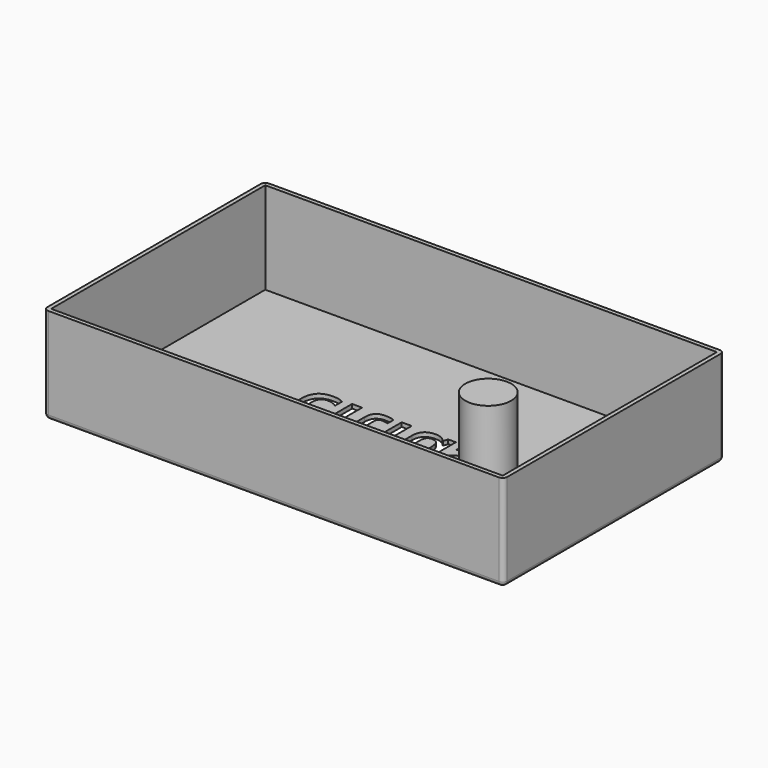
from build123d import *

# Parameters (mm, degrees)
F0_W         = 100
F0_H         = 60
F1_DEPTH     = 0.9
F2_W         = 98.2
F2_H         = 0.9
F3_DEPTH     = 20
F4_TEXT_SIZE = 14.6002053154
F5_DEPTH     = 2
F6_R         = 5
F7_DEPTH     = 25
F8_R         = 1
F8_2_R       = 1


# Not quite as in the source:
# - Text() gives the source's letters only with a copy of the font that has no kerning and outlines rounded to 1/6400 em; it was checked with that copy


with BuildPart() as f1:
    # F0 (on Top) → F1 (new body)
    with BuildSketch(Plane.XY):
        with Locations((2.3630317301, -8.3058337704)):
            Rectangle(F0_W, F0_H)
    extrude(amount=F1_DEPTH)

    # F2 (on face) → F3 (join)
    with BuildSketch(Plane.XY.offset(0.9)):
        Polygon((-46.7369682699, 21.6941662296), (-47.6369682699, 21.6941662296), (-47.6369682699, -38.3058337704), (-46.7369682699, -38.3058337704), (-46.7369682699, -37.4058337704), (-46.7369682699, 20.7941662296), align=None)
        Polygon((52.3630317301, 21.6941662296), (-46.7369682699, 21.6941662296), (-46.7369682699, 20.7941662296), (51.4630317301, 20.7941662296), (52.3630317301, 20.7941662296), align=None)
        with Locations((2.3630317301, -37.8558337704)):
            Rectangle(F2_W, F2_H)
        Polygon((52.3630317301, 20.7941662296), (51.4630317301, 20.7941662296), (51.4630317301, -37.4058337704), (51.4630317301, -38.3058337704), (52.3630317301, -38.3058337704), align=None)
    extrude(amount=F3_DEPTH)

    # F4 (on face) → F5 (cut)
    with BuildSketch(Plane(origin=(0, 0, 0), x_dir=(1, 0, 0), z_dir=(0, 0, -1))):
        with Locations((-17.6369682699, 2.7936859433)):
            Text('citius', F4_TEXT_SIZE, font='Open Sans', font_style=FontStyle.BOLD, text_align=(TextAlign.LEFT, TextAlign.BOTTOM))
    extrude(amount=-F5_DEPTH, mode=Mode.SUBTRACT)

    # F8
    f8_edges = [f1.edges().sort_by_distance(p)[0] for p in [
        (52.363032, 21.694166, 10.45),
        (52.363032, -38.305834, 10.45),
        (-47.636968, -38.305834, 10.45),
        (-47.636968, 21.694166, 10.45),
        (2.363032, 21.694166, 0),
        (-47.636968, -8.305834, 0),
        (2.363032, -38.305834, 0),
        (52.363032, -8.305834, 0),
    ]]
    fillet(f8_edges, radius=F8_R)


with BuildPart() as f7:
    # F6 (on face) → F7 (new body)
    with BuildSketch(Plane.XY.offset(0.9)):
        with Locations((36.381021142, -22.4892441183)):
            Circle(F6_R)
    extrude(amount=F7_DEPTH)

    # F8#2
    f8_2_edges = [f7.edges().sort_by_distance(p)[0] for p in [
        (31.381021, -22.489244, 0.9),
    ]]
    fillet(f8_2_edges, radius=F8_2_R)


solid = Compound([f1.part, f7.part])
